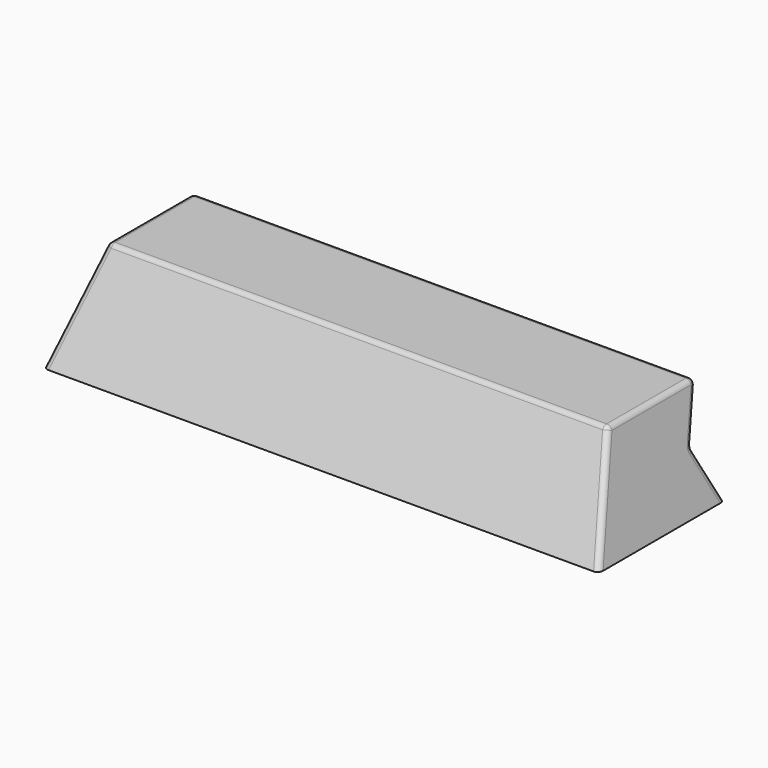
from build123d import *

# Parameters (mm, degrees)
F1_DEPTH = 25
F3_DEPTH = 14.1712295243
F4_R     = 0.5


with BuildPart() as f1:
    # F0 (on Right) → F1 (new body)
    with BuildSketch(Plane.YZ):
        Polygon((4.1702295243, 9.0889595507), (0, 0), (14.1702295243, 0), (12.0851147622, 4.5444797754), (14.1702295243, 9.0889595507), align=None)
    extrude(amount=F1_DEPTH)

    # F2 (on Front) → F3 (cut, through all)
    with BuildSketch(Plane.XZ):
        Polygon((22.5001233071, 9.0889595507), (25.0001233071, 0), (25.0001233071, 9.0889595507), align=None)
    extrude(amount=-F3_DEPTH, mode=Mode.SUBTRACT)

    # F4
    f4_edges = [f1.edges().sort_by_distance(p)[0] for p in [
        (11.250062, 14.17023, 9.08896),
        (11.875062, 12.085115, 4.54448),
        (22.500123, 9.17023, 9.08896),
        (23.125123, 13.127672, 6.81672),
        (23.750062, 2.085218, 4.544704),
        (11.250062, 4.17023, 9.08896),
        (24.375062, 13.127569, 2.272464),
    ]]
    fillet(f4_edges, radius=F4_R)

    # F5: F1 across face


with BuildPart() as f1_1:
    add(f1.part)
    add(f1.part.mirror(Plane(origin=(0, 7.5492536206, 4.2511231401), x_dir=(0, 1, 0), z_dir=(-1, 0, 0))))


solid = f1_1.part
